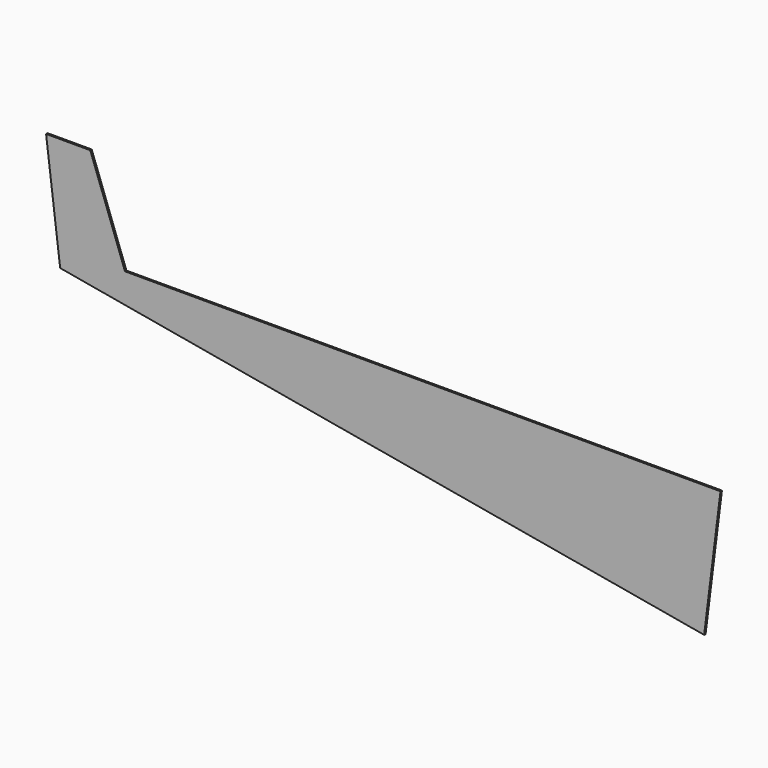
from build123d import *

# Parameters (mm, degrees)
F1_DEPTH = 4.7625


# Not quite as in the source:
# - a length typed as a fraction of an inch, garbled in the dataset ("3 / 203.2 mm" for 3/8 in), is restored


with BuildPart() as f1:
    # F0 (on Front) → F1 (new body)
    with BuildSketch(Plane.XZ):
        Polygon((1021.618930345, -309.1928088559), (1065.1506806603, 41.771382421), (-521.8711266779, 41.771382421), (-614.3195661815, 295.771382421), (-732.144496754, 295.771382421), (-694.6262103035, -6.7107132174), align=None)
    extrude(amount=F1_DEPTH)


solid = f1.part
